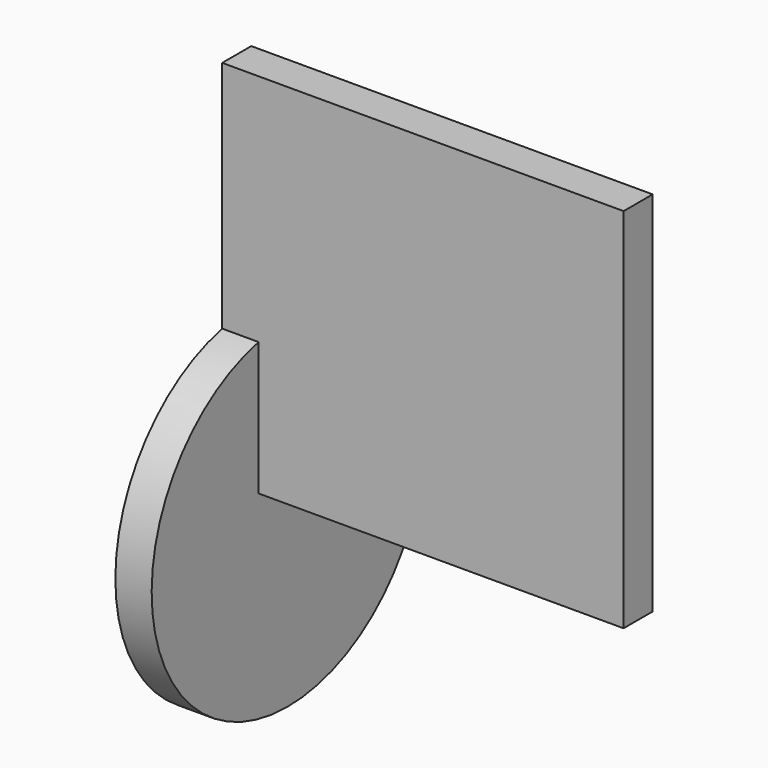
from build123d import *

# Parameters (mm, degrees)
F2_R     = 116.9838211005
F3_DEPTH = 25
F4_W     = 276.3622701168
F4_H     = 252.8828978539
F5_DEPTH = 25


# Not quite as in the source:
# - the program builds the solid bodies; features that only make, move or delete a surface that nothing else refers to are left out


with BuildPart() as f3:
    # F2 (on Right) → F3 (new body)
    with BuildSketch(Plane.YZ):
        Circle(F2_R)
    extrude(amount=F3_DEPTH)

    # F4 (on Front) → F5 (join)
    with BuildSketch(Plane.XZ):
        with Locations((138.1811350584, 148.9392518997)):
            Rectangle(F4_W, F4_H)
    extrude(amount=F5_DEPTH)


solid = f3.part
